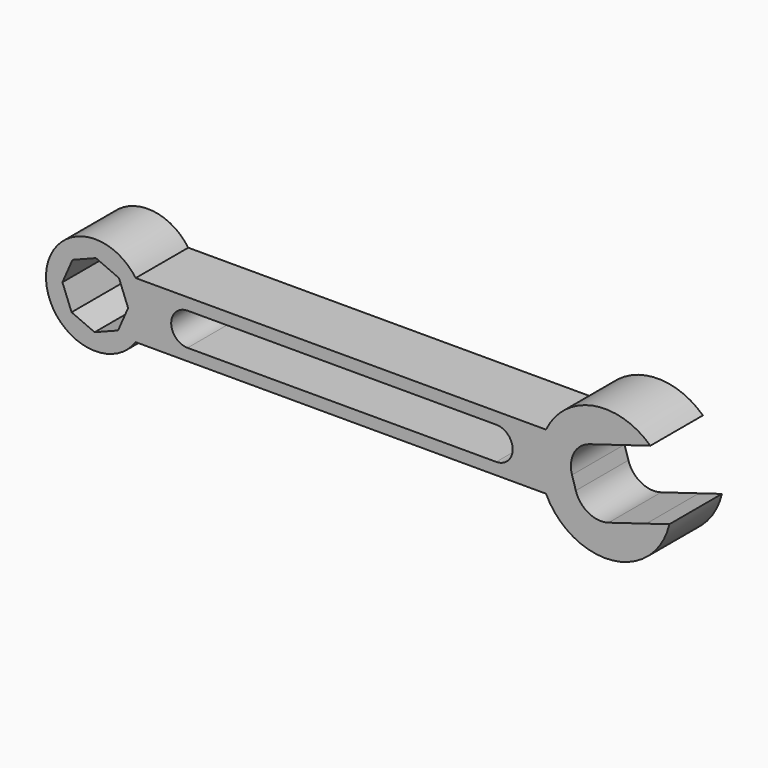
from build123d import *

# Parameters (mm, degrees)
F1_DEPTH = 25.4


# Not quite as in the source:
# - a feature of the source that left no trace in its solid (it failed there, or was rolled back) is left out


with BuildPart() as f1:
    # F0 (on Front) → F1 (new body)
    with BuildSketch(Plane.XZ):
        with BuildLine():
            ThreePointArc((-79.7143682919, -10.9044297796), (-77.1623604825, -5.7155262496), (-76.2847367633, 0))
            ThreePointArc((-76.2847367633, 0), (-77.1623604825, 5.7155262496), (-79.7143682919, 10.9044297796))
            ThreePointArc((-79.7143682919, 10.9044297796), (-114.3847367633, 0), (-79.7143682919, -10.9044297796))
        make_face()
        Polygon((-82.6373805848, -0.2591255978), (-86.5395795737, -9.1616161244), (-95.5938623611, -12.6973561785), (-104.4963528877, -8.7951571896), (-108.0320929418, 0.2591255978), (-104.1298939529, 9.1616161244), (-95.0756111655, 12.6973561785), (-86.1731206389, 8.7951571896), align=None, mode=Mode.SUBTRACT)
        with BuildLine():
            ThreePointArc((-79.7143682919, 10.9044297796), (-77.1623604825, 5.7155262496), (-76.2847367633, 0))
            ThreePointArc((-76.2847367633, 0), (-77.1623604825, -5.7155262496), (-79.7143682919, -10.9044297796))
            Line((-79.7143682919, -10.9044297796), (78.8772994949, -10.9044297796))
            ThreePointArc((78.8772994949, -10.9044297796), (76.4175133383, 0), (78.8772994949, 10.9044297796))
            Line((78.8772994949, 10.9044297796), (-79.7143682919, 10.9044297796))
        make_face()
        with BuildLine():
            ThreePointArc((-59.6665927425, -6.3275160443), (-65.9941087868, 0), (-59.6665927425, 6.3275160443))
            Line((-59.6665927425, 6.3275160443), (59.6665927425, 6.3275160443))
            ThreePointArc((59.6665927425, 6.3275160443), (65.9941087868, 0), (59.6665927425, -6.3275160443))
            Line((59.6665927425, -6.3275160443), (-59.6665927425, -6.3275160443))
        make_face(mode=Mode.SUBTRACT)
        with BuildLine():
            ThreePointArc((119.1980874489, 18.5223012497), (97.1020716916, 24.9584576863), (78.8772994949, 10.9044297796))
            ThreePointArc((78.8772994949, 10.9044297796), (76.4175133383, 0), (78.8772994949, -10.9044297796))
            ThreePointArc((78.8772994949, -10.9044297796), (104.5265574803, -25.2551198737), (126.5485838124, -5.7908680873))
            Line((126.5485838124, -5.7908680873), (117.6493461886, -8.4813364867))
            Line((117.6493461886, -8.4813364867), (103.0614445864, -12.8916343049))
            ThreePointArc((103.0614445864, -12.8916343049), (95.3234776063, -12.1222036637), (90.3959783062, -6.1065651155))
            Line((90.3959783062, -6.1065651155), (88.9258790335, -1.2439312481))
            ThreePointArc((88.9258790335, -1.2439312481), (89.6953096746, 6.494035732), (95.7109482229, 11.4215350322))
            Line((95.7109482229, 11.4215350322), (110.2988498251, 15.8318328503))
            Line((110.2988498251, 15.8318328503), (119.1980874489, 18.5223012497))
        make_face()
    extrude(amount=F1_DEPTH)


solid = f1.part
